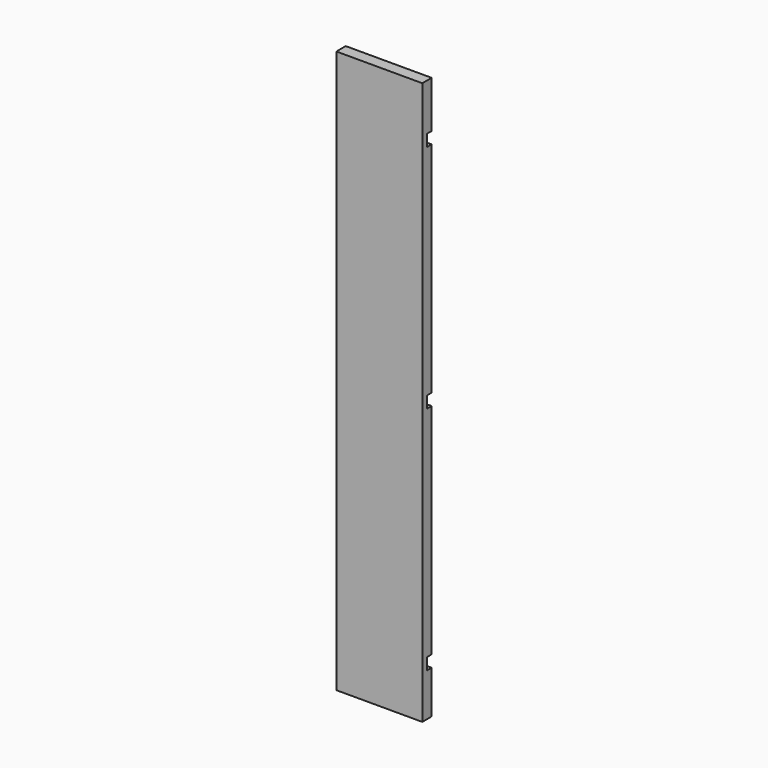
from build123d import *

# Parameters (mm, degrees)
F0_W     = 139.7
F0_H     = 914.4
F1_DEPTH = 19.05
F2_W     = 139.7
F2_H     = 19.05
F3_DEPTH = 9.525


# Not quite as in the source:
# - a length typed as a fraction of an inch, garbled in the dataset ("3 / 203.2 mm" for 3/8 in), is restored


with BuildPart() as f1:
    # F0 (on Front) → F1 (new body)
    with BuildSketch(Plane.XZ):
        Rectangle(F0_W, F0_H)
    extrude(amount=F1_DEPTH)

    # F2 (on face) → F3 (cut)
    with BuildSketch(Plane(origin=(0, 0, 0), x_dir=(-1, 0, 0), z_dir=(0, 1, 0))):
        with Locations((0, 371.475)):
            Rectangle(F2_W, F2_H)
        with Locations((0, -3.175)):
            Rectangle(F2_W, F2_H)
        with Locations((0, -377.825)):
            Rectangle(F2_W, F2_H)
    extrude(amount=-F3_DEPTH, mode=Mode.SUBTRACT)


solid = f1.part
